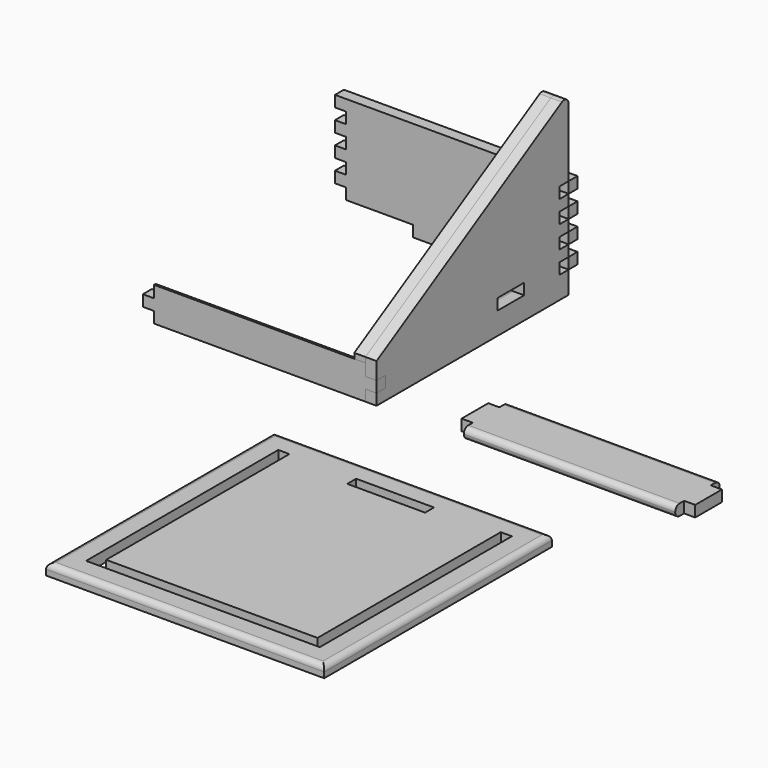
from build123d import *

# Parameters (mm, degrees)
F0_W      = 30
F0_H      = 10
F1_DEPTH  = 10
F3_W      = 5
F3_H      = 10.5
F4_DEPTH  = 250
F6_W      = 250
F6_H      = 255.863
F6_W_2    = 70
F6_H_2    = 10
F7_DEPTH  = 10
F9_DEPTH  = 190
F10_W     = 10
F10_H     = 10
F11_DEPTH = 10
F13_DEPTH = 10
F15_DEPTH = 10
F16_R     = 5
F16_2_R   = 5
F17_R     = 5
F18_R     = 4.99999


# Not quite as in the source:
# - a fillet or chamfer is up to 0.001 mm smaller than in the source, because OpenCascade refuses the exact size


with BuildPart() as f1:
    # F0 (on Right) → F1 (new body)
    with BuildSketch(Plane.YZ):
        Polygon((220.836477965, 150), (5, 25.3867513459), (5, 10), (15, 10), (15, 0), (5, 0), (5, -10), (220.836477965, -10), (220.836477965, 0), (220.836477965, 10), (210.836477965, 10), (210.836477965, 20), (220.836477965, 20), (220.836477965, 30), (210.836477965, 30), (210.836477965, 40), (220.836477965, 40), (220.836477965, 50), (210.836477965, 50), (210.836477965, 60), (220.836477965, 60), (220.836477965, 70), (210.836477965, 70), (210.836477965, 80), (220.836477965, 80), align=None)
        with Locations((155.836477965, 15)):
            Rectangle(F0_W, F0_H, mode=Mode.SUBTRACT)
    extrude(amount=F1_DEPTH)

    # F3 (on face) → F4 (cut)
    with BuildSketch(Plane(origin=(0, 230.5792637576, 133.125), x_dir=(1, 0, 0), z_dir=(0, -0.8660254038, -0.5))):
        with Locations((2.5, 9.2355715851)):
            Rectangle(F3_W, F3_H)
    extrude(amount=F4_DEPTH, mode=Mode.SUBTRACT)


with BuildPart() as f5_1:
    # F5: instance of F1
    add(f1.part.mirror(Plane.YZ))

    # F16#2
    f16_2_edges = [f5_1.edges().sort_by_distance(p)[0] for p in [
        (-5, 220.836478, 150),
    ]]
    fillet(f16_2_edges, radius=F16_2_R)


with BuildPart() as f7:
    # F6 (on Top) → F7 (new body)
    with BuildSketch(Plane.XY):
        with Locations((127.095540093, -228.4486843696)):
            Rectangle(F6_W, F6_H)
        Polygon((222.095540093, -120.5171843696), (232.095540093, -120.5171843696), (232.095540093, -336.3801843696), (222.992540093, -336.3801843696), (31.232540093, -336.3801843696), (22.095540093, -336.3801843696), (22.095540093, -120.5171843696), (32.095540093, -120.5171843696), (32.095540093, -326.3801843696), (222.095540093, -326.3801843696), align=None, mode=Mode.SUBTRACT)
        with Locations((127.095540093, -125.5171843696)):
            Rectangle(F6_W_2, F6_H_2, mode=Mode.SUBTRACT)
    extrude(amount=F7_DEPTH)

    # F17
    f17_edges = [f7.edges().sort_by_distance(p)[0] for p in [
        (2.09554, -228.448684, 10),
        (127.09554, -356.380184, 10),
        (252.09554, -228.448684, 10),
        (127.09554, -100.517184, 10),
    ]]
    fillet(f17_edges, radius=F17_R)


with BuildPart() as f9:
    # F8 (on face) → F9 (new body)
    with BuildSketch(Plane(origin=(0, 0, 0), x_dir=(0, -1, 0), z_dir=(-1, 0, 0))):
        Polygon((-15, -10), (-5, -10), (-5, 20.6698729811), (-6.8301270189, 20.6698729811), (-12.0801270189, 11.5766062413), (-15, 13.262395693), align=None)
    extrude(amount=F9_DEPTH)

    # F10 (on face) → F11 (join)
    with BuildSketch(Plane.XZ.offset(-5)):
        with Locations((5, 5)):
            Rectangle(F10_W, F10_H)
        with Locations((-195, 5)):
            Rectangle(F10_W, F10_H)
    extrude(amount=-F11_DEPTH)


with BuildPart() as f13:
    # F12 (on face) → F13 (new body)
    with BuildSketch(Plane(origin=(0, 220.836477965, 0), x_dir=(-1, 0, 0), z_dir=(0, 1, 0))):
        Polygon((0, 10), (0, 0), (60, 0), (60, -10), (95, -10), (130, -10), (130, 0), (190, 0), (190, 10), (200, 10), (200, 20), (190, 20), (190, 30), (200, 30), (200, 40), (190, 40), (190, 50), (200, 50), (200, 60), (190, 60), (190, 70), (200, 70), (200, 80), (95, 80), (-10, 80), (-10, 70), (0, 70), (0, 60), (-10, 60), (-10, 50), (0, 50), (0, 40), (-10, 40), (-10, 30), (0, 30), (0, 20), (-10, 20), (-10, 10), align=None)
    extrude(amount=F13_DEPTH)


with BuildPart() as f15:
    # F14 (on Top) → F15 (new body)
    with BuildSketch(Plane.XY):
        Polygon((292.7889656446, 37.0870450573), (102.7889656446, 37.0870450573), (102.7889656446, 27.0870450573), (92.7889656446, 27.0870450573), (92.7889656446, -2.9129549427), (102.7889656446, -2.9129549427), (102.7889656446, -12.9129549427), (292.7889656446, -12.9129549427), (292.7889656446, -2.9129549427), (302.7889656446, -2.9129549427), (302.7889656446, 27.0870450573), (292.7889656446, 27.0870450573), align=None)
    extrude(amount=F15_DEPTH)

    # F18 (radius 5 in the source; OpenCascade refuses exactly that, so slightly less here)
    f18_edges = [f15.edges().sort_by_distance(p)[0] for p in [
        (197.788966, 37.087045, 10),
        (197.788966, 37.087045, 0),
        (197.788966, -12.912955, 10),
        (197.788966, -12.912955, 0),
    ]]
    fillet(f18_edges, radius=F18_R)


with BuildPart() as f1_1:
    add(f1.part)

    # F16
    f16_edges = [f1_1.edges().sort_by_distance(p)[0] for p in [
        (5, 220.836478, 150),
    ]]
    fillet(f16_edges, radius=F16_R)


solid = Compound([f5_1.part, f7.part, f9.part, f13.part, f15.part, f1_1.part])
